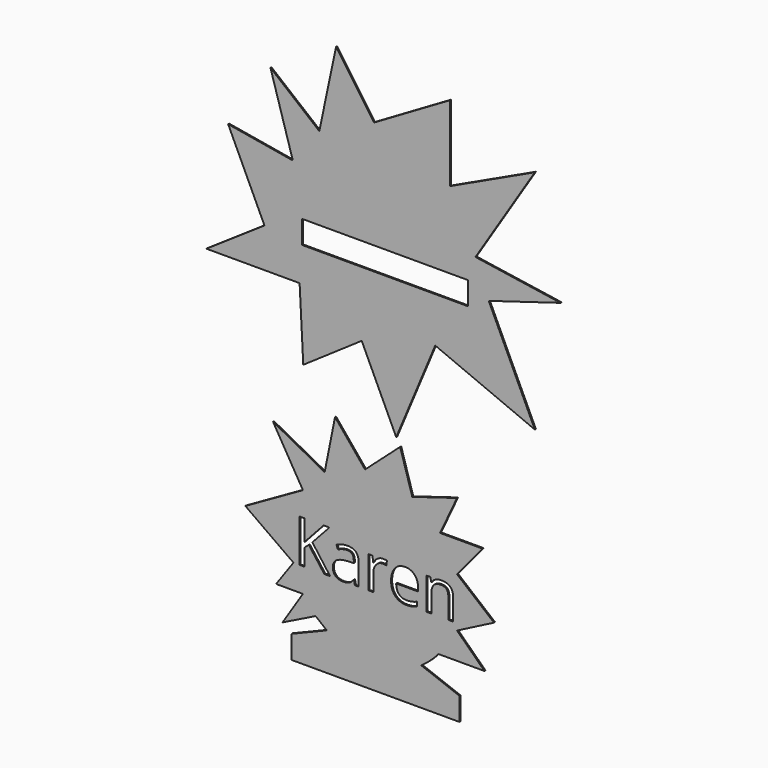
from build123d import *

# Parameters (mm, degrees)
F1_DEPTH = 0.25
F0_W     = 32.512
F0_H     = 4.5


# Not quite as in the source:
# - ends of sketch curves that miss each other by under 0.0002 mm in the source are joined


with BuildPart() as f1:
    # F0 (on Front) → F1 (new body)
    with BuildSketch(Plane.XZ):
        with BuildLine():
            Line((9.1908192262, -40.0406233966), (1.7421540068, -37.224151842))
            ThreePointArc((1.7421540068, -37.224151842), (3.5400615194, -35.8234885212), (5.1279398621, -34.1885660364))
            Line((5.1279398621, -34.1885660364), (14.1147730728, -34.1885660364))
            Line((14.1147730728, -34.1885660364), (8.7442151097, -28.9669632912))
            Line((8.7442151097, -28.9669632912), (15.9671846777, -25.2621360123))
            Line((15.9671846777, -25.2621360123), (8.7442151097, -19.2774161696))
            Line((8.7442151097, -19.2774161696), (13.7325850079, -13.2569432125))
            Line((13.7325850079, -13.2569432125), (5.4421929795, -13.2569432125))
            Line((5.4421929795, -13.2569432125), (8.7442151097, -6.1680306681))
            Line((8.7442151097, -6.1680306681), (0, -8.8137358894))
            Line((0, -8.8137358894), (-2.3697328302, -0.9816261545))
            Line((-2.3697328302, -0.9816261545), (-9.2416595929, -7.1157288558))
            Line((-9.2416595929, -7.1157288558), (-15.0963608176, 0))
            Line((-15.0963608176, 0), (-17.1216774215, -10.1288590574))
            Line((-17.1216774215, -10.1288590574), (-27.2082928568, -4.7430978157))
            Line((-27.2082928568, -4.7430978157), (-21.3730723744, -14.6107775405))
            Line((-21.3730723744, -14.6107775405), (-32.6230376959, -20.9873374552))
            Line((-32.6230376959, -20.9873374552), (-23.2184804045, -27.6845227927))
            Line((-23.2184804045, -27.6845227927), (-26.6130841116, -32.451412678))
            Line((-26.6130841116, -32.451412678), (-21.3730723744, -32.451412678))
            Line((-21.3730723744, -32.451412678), (-25.35588108, -38.6565104127))
            Line((-25.35588108, -38.6565104127), (-18.8906937658, -35.4634513731))
            Line((-18.8906937658, -35.4634513731), (-16.7138445578, -37.2174845321))
            Line((-16.7138445578, -37.2174845321), (-23.5751807738, -40.0406233966))
            Line((-23.5751807738, -40.0406233966), (-23.5751807738, -44.5406233966))
            Line((-23.5751807738, -44.5406233966), (9.1908192262, -44.5406233966))
            Line((9.1908192262, -44.5406233966), (9.1908192262, -40.0406233966))
        make_face()
        Polygon((-19.5294245035, -22.9701209884), (-16.0520058352, -27.6845227927), (-17.1922926493, -27.6845227927), (-20.2300167221, -23.6415218646), (-21.1039325364, -24.4169168982), (-21.1039325364, -27.6845227927), (-22.0727202137, -27.6845227927), (-22.0727202137, -19.3485700668), (-21.1039325364, -19.3485700668), (-21.1039325364, -23.4827939401), (-17.3236536903, -19.3485700668), (-16.1778934994, -19.3485700668), align=None, mode=Mode.SUBTRACT)
        with BuildLine():
            Line((-10.5038263124, -27.6845227927), (-11.2062429899, -27.6845227927))
            Line((-11.2062429899, -27.6845227927), (-11.3941622569, -26.7941868482))
            Line((-11.3941622569, -26.7941868482), (-11.4397737295, -26.7941868482))
            add(Edge.make_bspline(
                [(-11.4397737295, -26.7941868482), (-11.9068352085, -27.3816626149), (-12.3711599992, -27.5905631592)],
                knots=[0, 0, 0, 1, 1, 1], degree=2))
            add(Edge.make_bspline(
                [(-12.3711599992, -27.5905631592), (-12.8354847899, -27.7994637036), (-13.5324280907, -27.7994637036)],
                knots=[0, 0, 0, 1, 1, 1], degree=2))
            add(Edge.make_bspline(
                [(-13.5324280907, -27.7994637036), (-14.4610776721, -27.7994637036), (-14.988346295, -27.3196310122)],
                knots=[0, 0, 0, 1, 1, 1], degree=2))
            add(Edge.make_bspline(
                [(-14.988346295, -27.3196310122), (-15.5156149178, -26.8397983208), (-15.5156149178, -25.956760212)],
                knots=[0, 0, 0, 1, 1, 1], degree=2))
            add(Edge.make_bspline(
                [(-15.5156149178, -25.956760212), (-15.5156149178, -24.06479633), (-12.4888375984, -23.9735733849)],
                knots=[0, 0, 0, 1, 1, 1], degree=2))
            Line((-12.4888375984, -23.9735733849), (-11.428826976, -23.9389086657))
            Line((-11.428826976, -23.9389086657), (-11.428826976, -23.5502989195))
            add(Edge.make_bspline(
                [(-11.428826976, -23.5502989195), (-11.428826976, -22.8150419817), (-11.7444583662, -22.4647458724)],
                knots=[0, 0, 0, 1, 1, 1], degree=2))
            add(Edge.make_bspline(
                [(-11.7444583662, -22.4647458724), (-12.0600897563, -22.1144497631), (-12.7570330571, -22.1144497631)],
                knots=[0, 0, 0, 1, 1, 1], degree=2))
            add(Edge.make_bspline(
                [(-12.7570330571, -22.1144497631), (-13.5379014674, -22.1144497631), (-14.5231092748, -22.5924579956)],
                knots=[0, 0, 0, 1, 1, 1], degree=2))
            Line((-14.5231092748, -22.5924579956), (-14.8150226992, -21.8681478113))
            add(Edge.make_bspline(
                [(-14.8150226992, -21.8681478113), (-14.3534345969, -21.6181969416), (-13.8033602377, -21.4758891472)],
                knots=[0, 0, 0, 1, 1, 1], degree=2))
            add(Edge.make_bspline(
                [(-13.8033602377, -21.4758891472), (-13.2532858786, -21.3335813528), (-12.6986503722, -21.3335813528)],
                knots=[0, 0, 0, 1, 1, 1], degree=2))
            add(Edge.make_bspline(
                [(-12.6986503722, -21.3335813528), (-11.5820815239, -21.3335813528), (-11.0429539181, -21.8289219449)],
                knots=[0, 0, 0, 1, 1, 1], degree=2))
            add(Edge.make_bspline(
                [(-11.0429539181, -21.8289219449), (-10.5038263124, -22.3242625369), (-10.5038263124, -23.4189378785)],
                knots=[0, 0, 0, 1, 1, 1], degree=2))
            Line((-10.5038263124, -23.4189378785), (-10.5038263124, -27.6845227927))
        make_face(mode=Mode.SUBTRACT)
        with BuildLine():
            add(Edge.make_bspline(
                [(-6.7819301512, -21.6519494313), (-6.2911507064, -21.3208101405), (-5.7036749398, -21.3208101405)],
                knots=[0, 0, 0, 1, 1, 1], degree=2))
            add(Edge.make_bspline(
                [(-5.7036749398, -21.3208101405), (-5.28769831, -21.3208101405), (-4.9574712486, -21.3901395788)],
                knots=[0, 0, 0, 1, 1, 1], degree=2))
            Line((-4.9574712486, -21.3901395788), (-5.0888322896, -22.267704311))
            add(Edge.make_bspline(
                [(-5.0888322896, -22.267704311), (-5.4756175769, -22.1819547425), (-5.7730043781, -22.1819547425)],
                knots=[0, 0, 0, 1, 1, 1], degree=2))
            add(Edge.make_bspline(
                [(-5.7730043781, -22.1819547425), (-6.5319792815, -22.1819547425), (-7.0701946578, -22.7977096222)],
                knots=[0, 0, 0, 1, 1, 1], degree=2))
            add(Edge.make_bspline(
                [(-7.0701946578, -22.7977096222), (-7.6084100341, -23.4134645018), (-7.6084100341, -24.3311673298)],
                knots=[0, 0, 0, 1, 1, 1], degree=2))
            Line((-7.6084100341, -24.3311673298), (-7.6084100341, -27.6845227927))
            Line((-7.6084100341, -27.6845227927), (-8.5553042045, -27.6845227927))
            Line((-8.5553042045, -27.6845227927), (-8.5553042045, -21.4357510514))
            Line((-8.5553042045, -21.4357510514), (-7.7744357942, -21.4357510514))
            Line((-7.7744357942, -21.4357510514), (-7.66496826, -22.5924579956))
            Line((-7.66496826, -22.5924579956), (-7.6193567875, -22.5924579956))
            add(Edge.make_bspline(
                [(-7.6193567875, -22.5924579956), (-7.272709596, -21.9830887222), (-6.7819301512, -21.6519494313)],
                knots=[0, 0, 0, 1, 1, 1], degree=2))
        make_face(mode=Mode.SUBTRACT)
        with BuildLine():
            add(Edge.make_bspline(
                [(-0.0679213897, -27.7045918406), (-0.5149138209, -27.7994637036), (-1.14800106, -27.7994637036)],
                knots=[0, 0, 0, 1, 1, 1], degree=2))
            add(Edge.make_bspline(
                [(-1.14800106, -27.7994637036), (-2.5327653671, -27.7994637036), (-3.3346150548, -26.9547392317)],
                knots=[0, 0, 0, 1, 1, 1], degree=2))
            add(Edge.make_bspline(
                [(-3.3346150548, -26.9547392317), (-4.1364647425, -26.1100147598), (-4.1364647425, -24.6121340008)],
                knots=[0, 0, 0, 1, 1, 1], degree=2))
            add(Edge.make_bspline(
                [(-4.1364647425, -24.6121340008), (-4.1364647425, -23.0996575705), (-3.3920855102, -22.2102338555)],
                knots=[0, 0, 0, 1, 1, 1], degree=2))
            add(Edge.make_bspline(
                [(-3.3920855102, -22.2102338555), (-2.647706278, -21.3208101405), (-1.392478553, -21.3208101405)],
                knots=[0, 0, 0, 1, 1, 1], degree=2))
            add(Edge.make_bspline(
                [(-1.392478553, -21.3208101405), (-0.2193514786, -21.3208101405), (0.4648206098, -22.0934684858)],
                knots=[0, 0, 0, 1, 1, 1], degree=2))
            add(Edge.make_bspline(
                [(0.4648206098, -22.0934684858), (1.1489926983, -22.866126831), (1.1489926983, -24.1323013094)],
                knots=[0, 0, 0, 1, 1, 1], degree=2))
            Line((1.1489926983, -24.1323013094), (1.1489926983, -24.7307238294))
            Line((1.1489926983, -24.7307238294), (-3.1549058529, -24.7307238294))
            add(Edge.make_bspline(
                [(-3.1549058529, -24.7307238294), (-3.1257145104, -25.8308725477), (-2.5984458876, -26.4010159547)],
                knots=[0, 0, 0, 1, 1, 1], degree=2))
            add(Edge.make_bspline(
                [(-2.5984458876, -26.4010159547), (-2.0711772647, -26.9711593618), (-1.1133363409, -26.9711593618)],
                knots=[0, 0, 0, 1, 1, 1], degree=2))
            add(Edge.make_bspline(
                [(-1.1133363409, -26.9711593618), (-0.1044105678, -26.9711593618), (0.8807972396, -26.5497093553)],
                knots=[0, 0, 0, 1, 1, 1], degree=2))
            Line((0.8807972396, -26.5497093553), (0.8807972396, -27.3944338272))
            add(Edge.make_bspline(
                [(0.8807972396, -27.3944338272), (0.3790710414, -27.6097199777), (-0.0679213897, -27.7045918406)],
                knots=[0, 0, 0, 1, 1, 1], degree=2))
        make_face(mode=Mode.SUBTRACT)
        with BuildLine():
            Line((7.9870646651, -27.6845227927), (7.0401704947, -27.6845227927))
            Line((7.0401704947, -27.6845227927), (7.0401704947, -23.6415218646))
            add(Edge.make_bspline(
                [(7.0401704947, -23.6415218646), (7.0401704947, -22.8788980433), (6.6926110738, -22.5021472799)],
                knots=[0, 0, 0, 1, 1, 1], degree=2))
            add(Edge.make_bspline(
                [(6.6926110738, -22.5021472799), (6.3450516528, -22.1253965166), (5.6024968795, -22.1253965166)],
                knots=[0, 0, 0, 1, 1, 1], degree=2))
            add(Edge.make_bspline(
                [(5.6024968795, -22.1253965166), (4.6227624488, -22.1253965166), (4.1666477231, -22.6554018278)],
                knots=[0, 0, 0, 1, 1, 1], degree=2))
            add(Edge.make_bspline(
                [(4.1666477231, -22.6554018278), (3.7105329975, -23.185407139), (3.7105329975, -24.4059701448)],
                knots=[0, 0, 0, 1, 1, 1], degree=2))
            Line((3.7105329975, -24.4059701448), (3.7105329975, -27.6845227927))
            Line((3.7105329975, -27.6845227927), (2.7636388271, -27.6845227927))
            Line((2.7636388271, -27.6845227927), (2.7636388271, -21.4357510514))
            Line((2.7636388271, -21.4357510514), (3.533560484, -21.4357510514))
            Line((3.533560484, -21.4357510514), (3.6868150318, -22.2914222767))
            Line((3.6868150318, -22.2914222767), (3.7324265043, -22.2914222767))
            add(Edge.make_bspline(
                [(3.7324265043, -22.2914222767), (4.0243399287, -21.8298341743), (4.5488718632, -21.5753221574)],
                knots=[0, 0, 0, 1, 1, 1], degree=2))
            add(Edge.make_bspline(
                [(4.5488718632, -21.5753221574), (5.0734037977, -21.3208101405), (5.7174377903, -21.3208101405)],
                knots=[0, 0, 0, 1, 1, 1], degree=2))
            add(Edge.make_bspline(
                [(5.7174377903, -21.3208101405), (6.846777851, -21.3208101405), (7.4169212581, -21.8654111229)],
                knots=[0, 0, 0, 1, 1, 1], degree=2))
            add(Edge.make_bspline(
                [(7.4169212581, -21.8654111229), (7.9870646651, -22.4100121054), (7.9870646651, -23.6086816044)],
                knots=[0, 0, 0, 1, 1, 1], degree=2))
            Line((7.9870646651, -23.6086816044), (7.9870646651, -27.6845227927))
        make_face(mode=Mode.SUBTRACT)
    extrude(amount=F1_DEPTH)


with BuildPart() as f1b:
    # F0 (on Front) → F1, piece 2 (new body)
    with BuildSketch(Plane.XZ):
        Polygon((7.3384060524, 61.8007461503), (-7.4825045565, 53.1481337773), (-14.8905524984, 63.7956540063), (-18.1692637377, 48.1945759981), (-27.7149509639, 55.9998750687), (-23.3457159576, 41.4591850034), (-35.9800159931, 43.6025373638), (-28.8859348023, 28.4744197975), (-40.2339622378, 20.7956727132), (-22.0192076354, 20.7956727132), (-21.3027521968, 6.9821728393), (-9.8811194407, 14.8193339882), (-3.1387680301, 0.4413325464), (4.4895137118, 18.6819890642), (23.9580851048, 10.5401906836), (14.9421067908, 29.766559504), (28.9818804081, 33.9852774667), (12.348745206, 36.4689829807), (23.9580851048, 54.8162585276), (7.3384060524, 47.0278221128), align=None)
        with Locations((-5.3317387673, 29.766559504)):
            Rectangle(F0_W, F0_H, mode=Mode.SUBTRACT)
    extrude(amount=F1_DEPTH)


solid = Compound([f1.part, f1b.part])
